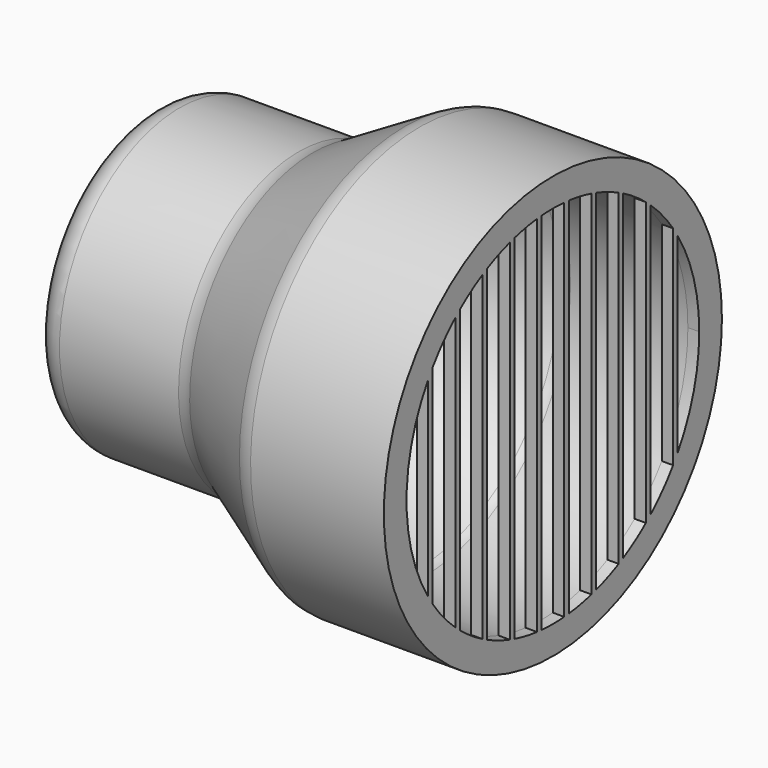
from build123d import *

# Parameters (mm, degrees)
F2_R     = 37.25
F3_DEPTH = 2
F5_DEPTH = 2
F6_R     = 4.99999
F7_R     = 3


# Not quite as in the source:
# - a fillet or chamfer is up to 0.001 mm smaller than in the source, because OpenCascade refuses the exact size


with BuildPart() as f1:
    # F0 (on Top) → F1 (revolve)
    with BuildSketch(Plane.XY):
        Polygon((-28.6666666667, 26.5), (-28.6666666667, 21.5), (0, 21.5), (18.6195461814, 32.25), (40.1195461814, 32.25), (40.1195461814, 37.25), (17.2798002192, 37.25), (-1.3397459622, 26.5), align=None)
    revolve(axis=Axis((-8.7595172226, 0, 0), (1, 0, 0)))

    # F2 (on face) → F3 (join)
    with BuildSketch(Plane.YZ.offset(40.1195461814)):
        Circle(F2_R)
    extrude(amount=F3_DEPTH)

    # F4 (on face) → F5 (cut, through all)
    with BuildSketch(Plane.YZ.offset(42.1195461814)):
        with BuildLine():
            ThreePointArc((32.25, 0), (31.0397930083, 8.7517855321), (27.5, 16.8467355888))
            Line((27.5, 16.8467355888), (27.5, -16.8467355888))
            ThreePointArc((27.5, -16.8467355888), (31.0397930083, -8.7517855321), (32.25, 0))
        make_face()
        with BuildLine():
            ThreePointArc((26.5, 18.3796762757), (24.1661621929, 21.3555403788), (21.5, 24.0377307581))
            Line((21.5, 24.0377307581), (21.5, -24.0377307581))
            ThreePointArc((21.5, -24.0377307581), (24.1661621929, -21.3555403788), (26.5, -18.3796762757))
            Line((26.5, -18.3796762757), (26.5, 18.3796762757))
        make_face()
        with BuildLine():
            ThreePointArc((20.5, 24.8960338207), (18.0793922843, 26.7057685647), (15.5, 28.2809564902))
            Line((15.5, 28.2809564902), (15.5, -28.2809564902))
            ThreePointArc((15.5, -28.2809564902), (18.0793922843, -26.7057685647), (20.5, -24.8960338207))
            Line((20.5, -24.8960338207), (20.5, 24.8960338207))
        make_face()
        with BuildLine():
            ThreePointArc((14.5, 28.806466288), (12.0421178111, 29.9173845552), (9.5, 30.8190282131))
            Line((9.5, 30.8190282131), (9.5, -30.8190282131))
            ThreePointArc((9.5, -30.8190282131), (12.0421178111, -29.9173845552), (14.5, -28.806466288))
            Line((14.5, -28.806466288), (14.5, 28.806466288))
        make_face()
        with BuildLine():
            ThreePointArc((8.5, 31.1096849872), (6.0187660071, 31.6833861156), (3.5, 32.0595149683))
            Line((3.5, 32.0595149683), (3.5, -32.0595149683))
            ThreePointArc((3.5, -32.0595149683), (6.0187660071, -31.6833861156), (8.5, -31.1096849872))
            Line((8.5, -31.1096849872), (8.5, 31.1096849872))
        make_face()
        with BuildLine():
            ThreePointArc((2.5, 32.1529547631), (0, 32.25), (-2.5, 32.1529547631))
            Line((-2.5, 32.1529547631), (-2.5, -32.1529547631))
            ThreePointArc((-2.5, -32.1529547631), (0, -32.25), (2.5, -32.1529547631))
            Line((2.5, -32.1529547631), (2.5, 32.1529547631))
        make_face()
        with BuildLine():
            Line((-3.5, -32.0595149683), (-3.5, 32.0595149683))
            ThreePointArc((-3.5, 32.0595149683), (-6.0187660071, 31.6833861156), (-8.5, 31.1096849872))
            Line((-8.5, 31.1096849872), (-8.5, -31.1096849872))
            ThreePointArc((-8.5, -31.1096849872), (-6.0187660071, -31.6833861156), (-3.5, -32.0595149683))
        make_face()
        with BuildLine():
            Line((-9.5, -30.8190282131), (-9.5, 30.8190282131))
            ThreePointArc((-9.5, 30.8190282131), (-12.0421178111, 29.9173845552), (-14.5, 28.806466288))
            Line((-14.5, 28.806466288), (-14.5, -28.806466288))
            ThreePointArc((-14.5, -28.806466288), (-12.0421178111, -29.9173845552), (-9.5, -30.8190282131))
        make_face()
        with BuildLine():
            Line((-15.5, -28.2809564902), (-15.5, 28.2809564902))
            ThreePointArc((-15.5, 28.2809564902), (-18.0793922843, 26.7057685647), (-20.5, 24.8960338207))
            Line((-20.5, 24.8960338207), (-20.5, -24.8960338207))
            ThreePointArc((-20.5, -24.8960338207), (-18.0793922843, -26.7057685647), (-15.5, -28.2809564902))
        make_face()
        with BuildLine():
            Line((-21.5, -24.0377307581), (-21.5, 24.0377307581))
            ThreePointArc((-21.5, 24.0377307581), (-24.1661621929, 21.3555403788), (-26.5, 18.3796762757))
            Line((-26.5, 18.3796762757), (-26.5, -18.3796762757))
            ThreePointArc((-26.5, -18.3796762757), (-24.1661621929, -21.3555403788), (-21.5, -24.0377307581))
        make_face()
        with BuildLine():
            Line((-27.5, -16.8467355888), (-27.5, 16.8467355888))
            ThreePointArc((-27.5, 16.8467355888), (-32.25, 0), (-27.5, -16.8467355888))
        make_face()
    extrude(amount=-F5_DEPTH, mode=Mode.SUBTRACT)

    # F6 (radius 5 in the source; OpenCascade refuses exactly that, so slightly less here)
    f6_edges = [f1.edges().sort_by_distance(p)[0] for p in [
        (-28.666667, -26.5, 0),
        (-1.339746, -26.5, 0),
        (17.2798, -37.25, 0),
    ]]
    fillet(f6_edges, radius=F6_R)

    # F7
    f7_edges = [f1.edges().sort_by_distance(p)[0] for p in [
        (18.619546, -32.25, 0),
        (0, -21.5, 0),
    ]]
    fillet(f7_edges, radius=F7_R)


solid = f1.part
